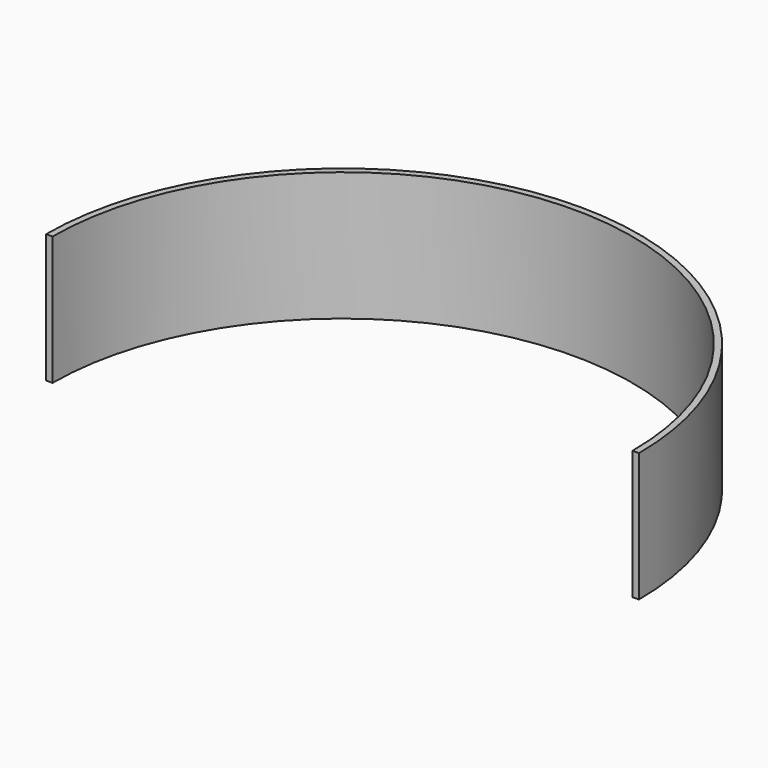
from build123d import *

# Parameters (mm, degrees)
F1_DEPTH = 20


with BuildPart() as f1:
    # F0 (on Top) → F1 (new body)
    with BuildSketch(Plane.XY):
        with BuildLine():
            ThreePointArc((-45, 0), (0, 45), (45, 0))
            Line((45, 0), (46, 0))
            ThreePointArc((46, 0), (0, 46), (-46, 0))
            Line((-46, 0), (-45, 0))
        make_face()
    extrude(amount=F1_DEPTH)


solid = f1.part
